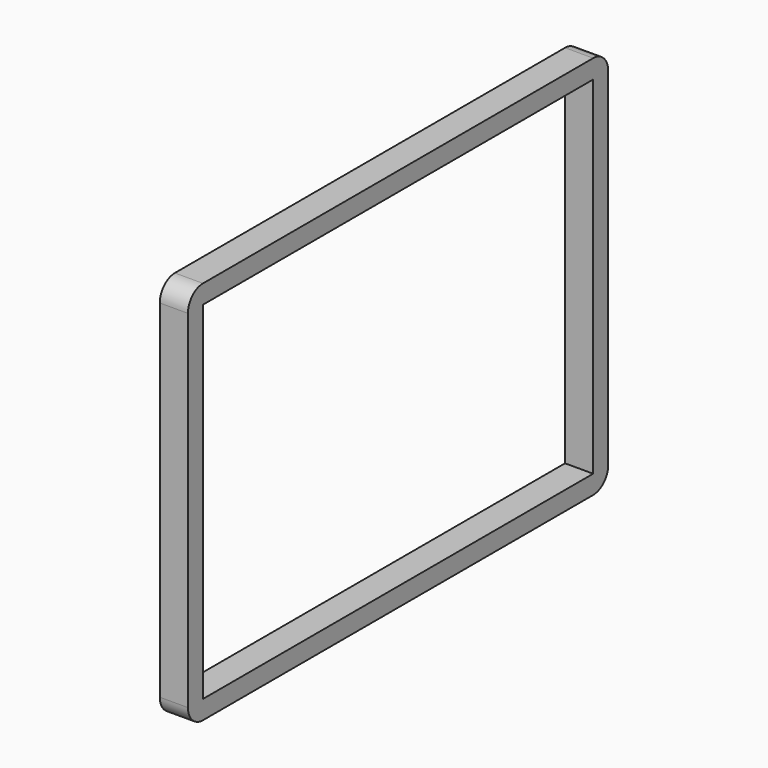
from build123d import *

# Parameters (mm, degrees)
F1_DEPTH = 9.525


# Not quite as in the source:
# - a length typed as a fraction of an inch, garbled in the dataset ("3 / 203.2 mm" for 3/8 in), is restored


with BuildPart() as f1:
    # F0 (on Right) → F1 (new body)
    with BuildSketch(Plane.YZ):
        with BuildLine():
            ThreePointArc((88.9, 58.7375), (87.0401280605, 63.2276280605), (82.55, 65.0875))
            Line((82.55, 65.0875), (-82.55, 65.0875))
            ThreePointArc((-82.55, 65.0875), (-87.0401280605, 63.2276280605), (-88.9, 58.7375))
            Line((-88.9, 58.7375), (-88.9, -58.7375))
            ThreePointArc((-88.9, -58.7375), (-87.0401280605, -63.2276280605), (-82.55, -65.0875))
            Line((-82.55, -65.0875), (82.55, -65.0875))
            ThreePointArc((82.55, -65.0875), (87.0401280605, -63.2276280605), (88.9, -58.7375))
            Line((88.9, -58.7375), (88.9, 58.7375))
        make_face()
        Polygon((82.55, 58.7375), (82.55, 53.975), (82.55, -53.975), (82.55, -58.7375), (74.6125, -58.7375), (-74.6125, -58.7375), (-82.55, -58.7375), (-82.55, -53.975), (-82.55, 53.975), (-82.55, 58.7375), (-74.6125, 58.7375), (74.6125, 58.7375), align=None, mode=Mode.SUBTRACT)
    extrude(amount=F1_DEPTH)


solid = f1.part
